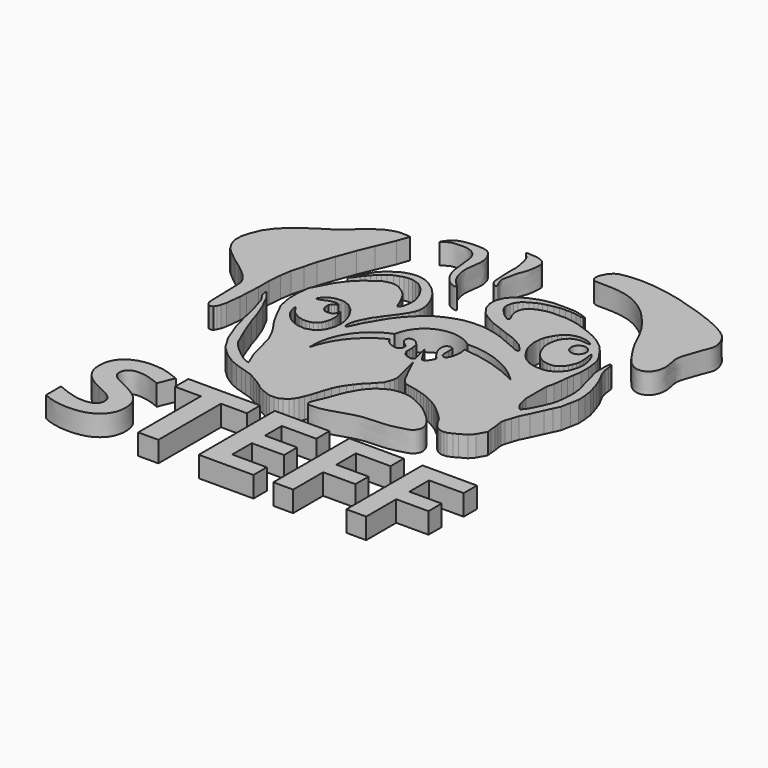
from build123d import *

# Parameters (mm, degrees)
F0_R         = 0.7148754106
F1_DEPTH     = 2
F2_TEXT_SIZE = 12.8132962143
F3_DEPTH     = 2


# Not quite as in the source:
# - Text() gives the source's letters only with a copy of the font that has no kerning and outlines rounded to 1/6400 em; it was checked with that copy


with BuildPart() as f1:
    # F0 (on Top) → F1 (new body)
    with BuildSketch(Plane.XY):
        Polygon((24.2907386273, 8.5276849568), (23.6116535962, 11.1627820879), (24.8693041503, 8.5963644087), (25.0527132303, 8.346952498), (25.2517424524, 8.1386491656), (25.4696086049, 8.0059850588), (25.712300092, 7.9455329105), (26.0382480919, 7.8855678439), (26.3718944043, 7.8116664663), (26.6574658453, 7.7494843863), (27.1523203701, 7.6115736738), (27.561949566, 7.478334941), (27.965053916, 7.3233088478), (28.3012557775, 7.1526789106), (28.7174619734, 6.9484477863), (29.083294794, 6.734599825), (29.4517893344, 6.4759417437), (29.7768972814, 6.1944676563), (30.1108527929, 5.9097232297), (30.4275006056, 5.6273424998), (30.7160790929, 5.3253171997), (30.9498113344, 5.0806938009), (31.1575550586, 4.7167097218), (31.3333831728, 4.4164536521), (31.5317050489, 4.1467623255), (31.7468166899, 3.954929697), (31.9705717266, 3.7988221738), (32.2670228779, 3.6963894963), (32.5457528234, 3.6963894963), (32.8103117645, 3.7337348331), (33.2356244326, 3.9057510439), (33.6025530184, 4.127406268), (34.2337685054, 4.4553116895), (34.6451625228, 4.9206055701), (35.1030383865, 5.7764222953), (35.0452120334, 6.2305437235), (35.0145325065, 6.7541487515), (34.9361580001, 7.2351241033), (34.886803478, 7.6227146201), (34.9578771205, 8.0304975484), (35.1350092745, 8.5627562235), (35.3541485965, 9.2212408781), (35.7608534396, 10.0460797548), (36.248870194, 11.1179118976), (36.5554206073, 11.7735937238), (36.8498107069, 12.3952152207), (37.0237194002, 13.3052840829), (37.1836354921, 14.1115276293), (37.134337691, 14.952889251), (37.0374396443, 15.7138481736), (36.8498107069, 16.3053733847), (36.6619750857, 16.906498), (36.4415954424, 17.4924607419), (36.1356697977, 18.0813653228), (35.888556391, 18.5570567846), (35.7323108402, 19.0970151623), (35.6707081445, 19.5807929325), (35.6309190392, 19.893264398), (35.5439911266, 20.0728083305), (35.3934951127, 20.0257822871), (35.3541485965, 18.992587924), (35.3976197821, 18.2506686842), (35.6607027352, 17.4087323248), (35.9177728508, 16.352175986), (36.1356697977, 15.6548470259), (36.2420044839, 14.8197803646), (36.2420044839, 14.1903264448), (36.1978299916, 13.4835708886), (36.0890701413, 12.796677649), (35.888556391, 12.194160372), (35.6456115842, 11.6420071572), (35.3640131652, 11.0622476786), (35.1376309991, 10.6370896101), (34.7761988164, 10.1604085924), (34.6406921744, 10.1180663332), (34.5081761479, 10.3389276192), (34.2337685054, 10.7001692558), (34.0774953365, 11.2002855167), (33.9554265588, 11.7979329079), (33.9554265588, 12.4641489238), (33.9554265588, 13.3207123727), (33.9554265588, 14.2623815543), (34.1256596148, 14.9280913174), (34.2337685054, 15.7283823937), (34.3045257032, 16.3797922432), (34.3799516559, 16.9626325369), (34.5074385405, 17.7104417235), (34.5074385405, 18.1742515415), (34.5074385405, 18.6049304903), (34.4467014074, 19.1184319556), (34.3787092705, 19.6089588158), (34.2337685054, 20.0728083305), (33.9935868979, 20.5351561308), (33.6651131511, 20.9820568562), (33.3983413875, 21.3733203709), (32.9359397292, 21.8890774995), (32.464645803, 22.2803428769), (31.9755636156, 22.6138047874), (31.4716597906, 22.8858546951), (30.7917307192, 23.1823699325), (30.0647059854, 23.4439208808), (29.4207148254, 23.6756000668), (28.7761632353, 23.8058827817), (28.0895289034, 23.8949786872), (27.538202703, 23.8949786872), (27.1113682538, 23.8949786872), (26.7201047391, 23.8949786872), (26.2932702899, 23.823838681), (25.8842222393, 23.7215775996), (25.4940543223, 23.5871449113), (25.1194797456, 23.3925599605), (24.8438157141, 23.1524650007), (24.6570762247, 22.9034796357), (24.5589371771, 22.509438917), (24.5589371771, 22.1156086773), (24.6831804903, 21.6857026522), (24.7969844564, 21.4666308677), (24.9062236398, 21.2563462555), (24.9062236398, 21.1131349206), (24.8109105975, 21.021023119), (24.6842466295, 21.0665911436), (24.4121458381, 21.242024377), (24.1257250309, 21.4711613953), (23.8249823451, 21.7719040811), (23.5651400528, 22.0967382025), (23.3939066529, 22.4263612181), (23.3939066529, 22.7287001908), (23.4363881231, 23.0534564958), (23.5403869301, 23.342538625), (23.7226802856, 23.6493237317), (23.9805597812, 23.8983109593), (24.382356189, 24.1568095487), (24.6950193107, 24.3192325799), (24.9631647021, 24.4585294276), (25.3410916775, 24.5830230415), (25.7301535457, 24.6850401163), (26.2492913753, 24.7960276902), (26.746949181, 24.8712133616), (27.2768270224, 24.8998552561), (27.8496704996, 24.8998552561), (28.3222645521, 24.8568914831), (28.8235023618, 24.7540798282), (29.1257899468, 24.7540798282), (29.1638504714, 24.8598754406), (28.5766869783, 25.0711105764), (27.9537215829, 25.2035818994), (27.3271705955, 25.2300128341), (26.6277603805, 25.2300128341), (25.8872099221, 25.2300128341), (25.2358000726, 25.1134447753), (24.6392469853, 24.9557346106), (23.9192657173, 24.6677435935), (23.3912821859, 24.3934653699), (22.904438898, 23.9957626909), (22.5187186152, 23.5871449113), (22.1901535988, 22.8337235749), (22.1901535988, 22.1508350223), (22.3913134389, 21.4811542993), (22.9124389589, 20.7325294614), (23.5034003854, 20.312288776), (24.3307463825, 19.8657847941), (25.2762846649, 19.5112079382), (26.195557788, 19.1566310823), (27.1148309112, 18.8414528966), (28.0735008419, 18.2898882776), (28.6644622684, 17.6595300436), (28.6644622684, 17.4625422806), (28.4018144011, 17.4625422806), (28.0341040343, 17.6332648844), (27.5876000524, 17.8302526474), (26.9703734666, 18.0797688663), (26.3925455511, 18.3424185961), (25.65712668, 18.605068326), (24.8166490346, 18.7889225781), (24.1206269711, 18.8939832151), (23.2276190072, 18.8939832151), (22.3477426916, 18.7889225781), (21.5991921723, 18.5788031667), (20.942568779, 18.3161534369), (20.2356303337, 17.9612244696), (19.5574704558, 17.4891503396), (18.94024387, 16.8775692582), (18.3886792511, 16.29973948), (17.8765133023, 15.6431160867), (17.3677299172, 14.8263750598), (17.0370518032, 14.2229637131), (16.7094636708, 13.7018356472), (16.4351854473, 13.0847096443), (16.2500478327, 12.7144344151), (16.1197669804, 12.5061682631), (15.9746445923, 12.5061682631), (15.9414857626, 12.6047236845), (15.9414857626, 12.9818553105), (16.0437058657, 13.4173221886), (16.1877013743, 13.8561669737), (16.434552148, 14.3018681556), (16.6196897626, 14.699571766), (16.9143974781, 15.0882480666), (17.1527792951, 15.4448095709), (17.4903795123, 15.904225409), (17.8496371955, 16.4013300091), (18.1257128716, 16.793359071), (18.3797031641, 17.1909090132), (18.60056445, 17.616065219), (18.7287908047, 18.0798731744), (18.7287908047, 18.5411386192), (18.6502356082, 19.0139841288), (18.4901729226, 19.4897260517), (18.3062069118, 19.9071634561), (18.0687734729, 20.3393351903), (17.7815575153, 20.7519363612), (17.461432144, 21.1076308042), (17.1032305807, 21.4480049908), (16.6780743748, 21.7516887933), (16.3688678294, 21.9559855759), (15.9713178873, 22.1326742321), (15.5075099319, 22.2375839949), (15.1099609211, 22.2872775048), (14.6461520344, 22.2431048751), (14.1713013873, 22.1326742321), (13.7847941369, 21.9780709594), (13.3872451261, 21.7461679131), (13.0614750087, 21.5087421238), (12.6804895699, 21.2050583214), (12.3034892604, 20.8377465606), (11.8868350983, 20.1465655118), (11.5168923512, 19.516505301), (11.1311545422, 18.8449039694), (11.2187303603, 18.771706149), (11.5279359743, 19.1416479647), (11.7989871651, 19.516505301), (12.0384553447, 19.8146682233), (12.3034892604, 20.1349165291), (12.6182157546, 20.4662084579), (12.9119114889, 20.7217949708), (13.2593411217, 20.9636443443), (13.6547806244, 21.2389138865), (14.1084849047, 21.4004018793), (14.4286891446, 21.5143729001), (14.8372817785, 21.5640664101), (15.201702714, 21.5640664101), (15.5661236495, 21.4702002704), (15.9802380949, 21.3155969977), (16.3897592574, 21.0091285408), (16.6838439588, 20.6882080435), (16.9931514671, 20.243871172), (17.249884792, 19.776975354), (17.4682307988, 19.008398056), (17.4682307988, 18.3950569481), (17.3413343728, 17.7605655044), (17.1527792951, 17.5220274957), (17.0370518032, 17.4891503396), (16.912657733, 17.667849112), (16.7705746947, 18.0670347203), (16.5224865601, 18.5686041272), (16.1992479116, 19.1564466804), (15.7762542367, 19.5794403553), (15.3321102262, 19.8755376041), (15.0360139087, 20.0447347015), (14.6341696382, 20.1482789205), (14.2209337805, 20.1482789205), (13.6408779873, 19.9834902043), (13.1381272476, 19.6335201961), (12.4223483726, 19.1352590919), (11.7989871651, 18.5574293137), (11.3192200661, 17.9664678872), (10.8595835045, 17.2967128456), (10.4262121022, 16.4562352002), (9.9797081202, 15.6420208514), (9.8468763754, 14.5015092567), (9.8468763754, 13.4440232068), (10.0920091452, 12.1402390962), (10.7457740232, 10.8184972778), (11.3288797438, 9.7580598667), (11.7989871651, 9.0827252716), (12.2325560078, 8.4165092558), (12.7189997584, 7.4330470525), (12.9833715037, 6.5024592914), (13.2265929133, 5.5824466981), (13.4197808802, 4.750484135), (14.0289058909, 3.304582322), (13.333641924, 3.6060682032), (12.6691423357, 4.0982901119), (11.9061982259, 4.750484135), (11.3293491304, 5.4122628644), (10.6122841348, 7.0427347797), (9.9340314046, 8.8061923161), (9.6277336048, 9.7929947206), (9.1117341071, 11.1345937476), (8.4279282019, 12.4762374908), (7.9319133823, 13.1022745853), (7.804713212, 13.1167639047), (7.9449221191, 12.5772664323), (8.3759939298, 11.9222681969), (8.862381801, 10.3419721127), (9.1928914189, 8.8791605085), (9.5785651356, 7.4076233432), (10.3000886738, 5.5316616781), (11.0682053491, 4.2288983241), (11.9425226003, 3.3970240038), (12.8638958558, 2.7919441927), (13.5361524299, 2.491829684), (14.148385264, 2.2997565102), (14.6885914728, 2.1316925995), (15.3428409249, 1.9216125365), (15.8410295844, 1.651509665), (16.4112485945, 1.3093793532), (16.901128231, 0.9802823328), (17.2268431634, 0.7096152985), (17.7006591111, 0.48602483), (18.159776926, 0.2906816371), (18.5862127692, 0.1488179405), (19.0066304058, 0.1488179405), (19.4182936102, 0.204862401), (19.7184178978, 0.3563134233), (20.102272972, 0.6089386869), (20.3555040061, 0.9136715089), (20.5445941538, 1.2202296639), (20.7265391946, 1.66916952), (20.9399685264, 2.1973256953), (21.1050435901, 2.7211178094), (21.302357316, 3.3580199815), (21.5112250298, 3.9624199271), (21.7900946736, 4.5490162447), (22.103626281, 5.0381072797), (22.4218014628, 5.4770857096), (22.8315256536, 5.9701390564), (23.2227928936, 6.3579040579), (23.6271154135, 6.7892442457), (23.9983685315, 7.2086052969), (24.1765435785, 7.6831914485), (24.2907386273, 8.0683119595), align=None)
        Polygon((11.4993210882, 14.6436599655), (11.4807495847, 14.6839478984), (11.7608709261, 15.1338391006), (12.1343657374, 15.3884943575), (12.6351881772, 15.5667532235), (13.1190326065, 15.6091963872), (13.5179935023, 15.5667532235), (13.9678847045, 15.3884952888), (14.2989363521, 15.1338391006), (14.6214999259, 14.8409856483), (14.8464459926, 14.5269101486), (15.1265664026, 14.0600418672), (15.2963371947, 13.6525938287), (15.4321538284, 13.1984576583), (15.5191710219, 12.5772664323), (15.4321538284, 11.9066741318), (15.2305616066, 11.2955011427), (14.9249751121, 10.8371209353), (14.4478578531, 10.4954016644), (13.8052644282, 10.303223896), (13.1184505299, 10.3686060756), (12.5454757363, 10.5638420209), (12.1337827295, 10.8184972778), (11.7608709261, 11.1570615731), (11.4165032282, 11.5569978952), (11.234426235, 11.9939806813), (11.1311545422, 12.3392948731), (11.1311545422, 12.6277012751), (11.3157930783, 12.3699041891), (11.4410180856, 12.1611954273), (11.5607800518, 11.9939806813), (11.7608709261, 11.8123194273), (11.9937377027, 11.6682782417), (12.1969040271, 11.5426084545), (12.4516179785, 11.4302448928), (12.7757415175, 11.3492142409), (13.1388790905, 11.3252056763), (13.4509988129, 11.3702220842), (13.7762400245, 11.4674906336), (14.0457884462, 11.6605456706), (14.2312953249, 11.9074266404), (14.3693480641, 12.1925352141), (14.4478578531, 12.4922143295), (14.5048173144, 12.8190219402), (14.5048173144, 13.1246084347), (14.4478578531, 13.4301949292), (14.3632018443, 13.7132630232), (14.2473119399, 14.1007692949), (14.2034748569, 13.9395063743), (14.1482995823, 13.7230493128), (13.9678847045, 13.5243312602), (13.7666308612, 13.4404751088), (13.4869674221, 13.4246200323), (13.2450452074, 13.4755503386), (13.0654336696, 13.5866501668), (12.9474079253, 13.7833601329), (12.8560017639, 14.0889990152), (12.8560017639, 14.3917575479), (12.9880212729, 14.6051892645), (13.1649551913, 14.7668998688), (13.3470012526, 14.8213436345), (13.492080383, 14.8213436345), (13.3693711012, 14.9926734984), (13.2219772786, 15.0340022519), (12.9998922348, 15.0340022519), (12.7477962524, 15.0340022519), (12.5125863395, 14.9636589922), (12.2378331184, 14.8491779601), (11.8866462507, 14.7028494296), (11.6887317845, 14.6436599655), align=None, mode=Mode.SUBTRACT)
        with BuildLine():
            ThreePointArc((21.2132986635, 12.1578685939), (20.4473145006, 12.3519211299), (19.9188143015, 12.9393525422))
            ThreePointArc((19.9188143015, 12.9393525422), (17.4443393612, 10.9808286692), (16.0302296281, 8.1596346572))
            Line((16.0302296281, 8.1596346572), (16.0302296281, 8.8887438178))
            ThreePointArc((16.0302296281, 8.8887438178), (17.1309249273, 11.8998701151), (19.6871741574, 13.8348123865))
            ThreePointArc((19.6871741574, 13.8348123865), (21.7523585958, 16.4088665275), (25.0181499869, 15.9341581166))
            ThreePointArc((25.0181499869, 15.9341581166), (28.3436366182, 15.3365141693), (31.1502087861, 13.4552400559))
            ThreePointArc((31.1502087861, 13.4552400559), (28.3497777615, 14.5861581292), (25.3769401461, 15.1187237352))
            ThreePointArc((25.3769401461, 15.1187237352), (25.4422622613, 14.1382532612), (25.1048468053, 13.2153555751))
            Line((25.1048468053, 13.2153555751), (24.8670708388, 13.2130132988))
            Line((24.8670708388, 13.2130132988), (24.6725827456, 13.3162793097))
            Line((24.6725827456, 13.3162793097), (24.6054362506, 13.559114188))
            Line((24.6054362506, 13.559114188), (24.6054362506, 13.7894693762))
            Line((24.6054362506, 13.7894693762), (24.6054362506, 14.1558581963))
            Line((24.6054362506, 14.1558581963), (24.526713416, 14.7497151047))
            Line((24.526713416, 14.7497151047), (24.2627672851, 14.822665602))
            Line((24.2627672851, 14.822665602), (23.9884052426, 14.7470263764))
            Line((23.9884052426, 14.7470263764), (23.8182302564, 14.4827486947))
            Line((23.8182302564, 14.4827486947), (23.8182302564, 14.0603547916))
            Line((23.8182302564, 14.0603547916), (23.9779874682, 13.5713601485))
            Line((23.9779874682, 13.5713601485), (24.3312194943, 13.0185233429))
            Line((24.3312194943, 13.0185233429), (24.523390457, 12.8111243248))
            Line((24.523390457, 12.8111243248), (24.6403124183, 12.662248686))
            Line((24.6403124183, 12.662248686), (24.6241055429, 12.5214504078))
            Line((24.6241055429, 12.5214504078), (24.4701392949, 12.2323455289))
            Line((24.4701392949, 12.2323455289), (24.3034362793, 11.9946226478))
            Line((24.3034362793, 11.9946226478), (24.1066366434, 11.8316644803))
            Line((24.1066366434, 11.8316644803), (23.8820519298, 11.8430582806))
            Line((23.8820519298, 11.8430582806), (22.9702237631, 13.3162793097))
            Line((22.9702237631, 13.3162793097), (23.3807861805, 11.7220170796))
            Line((23.3807861805, 11.7220170796), (23.2279766351, 11.4827072248))
            Line((23.2279766351, 11.4827072248), (22.9779239744, 11.5112746134))
            Line((22.9779239744, 11.5112746134), (22.7324981242, 11.5678431466))
            Line((22.7324981242, 11.5678431466), (22.4511884153, 11.7069706321))
            Line((22.4511884153, 11.7069706321), (22.2798530012, 11.911990121))
            Line((22.2798530012, 11.911990121), (22.1501979977, 12.1550420299))
            Line((22.1501979977, 12.1550420299), (22.1571419388, 12.5495754182))
            Line((22.1571419388, 12.5495754182), (22.1571419388, 12.8817595541))
            Line((22.1571419388, 12.8817595541), (22.0159050077, 13.5255521163))
            Line((22.0159050077, 13.5255521163), (21.7704791576, 13.7960957363))
            Line((21.7704791576, 13.7960957363), (21.4602295309, 13.9741916209))
            Line((21.4602295309, 13.9741916209), (21.1522914469, 13.9951081946))
            Line((21.1522914469, 13.9951081946), (20.9300220013, 13.8493236154))
            Line((20.9300220013, 13.8493236154), (20.8744574338, 13.5989040136))
            Line((20.8744574338, 13.5989040136), (20.9601242095, 13.3466133848))
            Line((20.9601242095, 13.3466133848), (21.138401702, 13.1408013403))
            Line((21.138401702, 13.1408013403), (21.4046649635, 12.9534667358))
            Line((21.4046649635, 12.9534667358), (21.5806290507, 12.7594145015))
            Line((21.5806290507, 12.7594145015), (21.5806290507, 12.4768838286))
            Line((21.5806290507, 12.4768838286), (21.4347653091, 12.2795756906))
            Line((21.4347653091, 12.2795756906), (21.2132986635, 12.1578685939))
        make_face(mode=Mode.SUBTRACT)
        Polygon((32.2024236749, 21.6673035175), (32.179441303, 21.6673035175), (31.8553186953, 21.6673035175), (31.6520147026, 21.7021815479), (31.3518978655, 21.7141862959), (31.1253126711, 21.6976795346), (30.8672133833, 21.6466598213), (30.6331254542, 21.5551257133), (30.4485540837, 21.4485842735), (30.3285084665, 21.3360413909), (30.1994588226, 21.196488291), (30.0794132054, 21.0584364831), (29.9531836063, 20.8845473826), (29.876653105, 20.7029785961), (29.8181306571, 20.5034017563), (29.7716129571, 20.3068275005), (29.7296587378, 20.0684703887), (29.7101512551, 19.8403839022), (29.7101512551, 19.6099672467), (29.7312997282, 19.3923842162), (29.7497604042, 19.2497763783), (29.7910254449, 19.1034711897), (29.8382937908, 18.9721714705), (29.9531836063, 18.6746716499), (30.0661027431, 18.4345804155), (30.2242137853, 18.1606703597), (30.3860846907, 17.9432407022), (30.5855646729, 17.7480056882), (30.8105107397, 17.5527688116), (31.0566779226, 17.4084641039), (31.3004666664, 17.3057081451), (31.5968194016, 17.2535458766), (31.9516181814, 17.2232011107), (32.3257111013, 17.2768924385), (32.6243907518, 17.4493014094), (32.8647308052, 17.6673643291), (33.0939218402, 17.9771948606), (33.227863254, 18.2949711665), (33.362194065, 18.6136713179), (33.4231950064, 18.9602397545), (33.4231950064, 19.3628575653), (33.3946980536, 19.708763808), (33.3308726549, 20.182909444), (33.3308726549, 20.4860251397), (33.4231950064, 20.3599780798), (33.6099788547, 20.0838726014), (33.7690375745, 19.708763808), (33.8740795851, 19.3726010621), (33.9617356658, 18.7977515161), (33.914945481, 18.2506686842), (33.7690375745, 17.6800843328), (33.6076992835, 17.2973088741), (33.3014242351, 16.8933086097), (33.0149382353, 16.6641175747), (32.6690301299, 16.4476614445), (32.3837674713, 16.3267005017), (32.0691242814, 16.2773840129), (31.7510031164, 16.263877973), (31.4508862793, 16.263877973), (31.1807841063, 16.2998922169), (30.9116253781, 16.3472679559), (30.6050814688, 16.4384189993), (30.3304772824, 16.5839754045), (30.1233995706, 16.708523035), (29.9004749988, 16.8775235037), (29.7210048884, 17.0521531254), (29.5469388366, 17.2532293946), (29.3863769621, 17.470812425), (29.2678326368, 17.6523812115), (29.1584187551, 17.8419287727), (29.0295065137, 18.0652551057), (28.9070916571, 18.3539465347), (28.8274753839, 18.6846721917), (28.7764556706, 19.0177988261), (28.7404414266, 19.2668940872), (28.7404414266, 19.5399969816), (28.7760427729, 19.9562570463), (28.8724050523, 20.3330893235), (28.9996804032, 20.6350503802), (29.1660893708, 20.9401287138), (29.3881744146, 21.2942622602), (29.6012554318, 21.5373560786), (29.8684542652, 21.7686625684), (30.1711949092, 21.9434156953), (30.5605319106, 22.0650732611), (31.0262441635, 22.1273452044), (31.4108729362, 22.0767054707), (31.7305819401, 21.9949505622), (32.1111753583, 21.8178052455), align=None, mode=Mode.SUBTRACT)
        with Locations((32.1084111929, 20.4434879124)):
            Circle(F0_R, mode=Mode.SUBTRACT)
    extrude(amount=F1_DEPTH)


with BuildPart() as f1b:
    # F0 (on Top) → F1, piece 2 (new body)
    with BuildSketch(Plane.XY):
        with BuildLine():
            add(Edge.make_bspline(
                [(21.6533839703, 0.9376612725), (21.5461532449, 1.1311018136), (22.0344466379, 2.0685321705), (22.4233865431, 3.1960527643), (22.7976823898, 4.1928911727), (23.4322410303, 5.3064863476), (24.0741523461, 5.9862297193), (24.9213836542, 6.4999262835), (25.5587741255, 6.7000867161), (26.749762737, 6.7702439862), (27.9176928338, 6.2376283208), (28.8198512588, 5.7654688033), (29.6107819403, 5.0857277809), (30.2381366471, 4.5356280251), (30.7263070916, 3.8476718611), (30.9750342426, 3.1452677218), (30.5835102235, 2.3943301946), (29.710791279, 2.1818872726), (28.6218613791, 1.895754702), (27.3538366614, 1.8417881518), (26.2622725948, 1.8209466564), (25.1013141845, 1.4925906791), (24.2392848072, 1.2327041384), (23.160959641, 0.8574094608), (22.3444714616, 0.790687727), (21.7348617966, 0.7906780755), (21.6533839703, 0.9376612725)],
                knots=[0, 0, 0, 0, 0.0438321528, 0.0917117069, 0.134904964, 0.1818612444, 0.2228157202, 0.2634959627, 0.2977575359, 0.3425918062, 0.3900760191, 0.4325789289, 0.4749537877, 0.5133887574, 0.5515986715, 0.5867264002, 0.6223953051, 0.6611041658, 0.7059206258, 0.7530279547, 0.7971544854, 0.8425262759, 0.8828675863, 0.9269997768, 0.9666947274, 1, 1, 1, 1], degree=3))
        make_face()
    extrude(amount=F1_DEPTH)


with BuildPart() as f1c:
    # F0 (on Top) → F1, piece 3 (new body)
    with BuildSketch(Plane.XY):
        Polygon((10.3225391358, 25.7849916816), (10.7130110264, 26.9054751843), (10.3810051279, 26.9496183768), (9.9722283454, 26.9686307203), (9.4923535362, 26.9548874348), (8.9554619044, 26.7985071987), (8.3642359823, 26.5584159642), (7.6800277457, 26.0781962425), (6.9777597673, 25.531988591), (6.3415174372, 24.9197557569), (5.6360246401, 24.3455377762), (4.846948199, 23.8633528352), (3.1822551973, 22.7532535791), (2.4919921998, 22.1590269357), (1.8679589467, 21.5046327781), (1.3222009086, 20.7276864662), (1.0364311747, 20.0472828001), (0.8728378755, 19.5575063688), (0.7451109813, 19.0589597071), (0.7146475837, 18.4794794768), (0.7926773396, 18.0983357131), (0.9277287754, 17.6481641829), (1.3414554996, 16.9711168855), (1.8028729828, 16.5448077023), (2.7450982016, 15.7723538578), (3.6151711829, 15.1611799374), (4.1467333212, 14.729898423), (4.5541818254, 14.3946027383), (4.9276766367, 14.0041308478), (5.2290190943, 13.6051708832), (5.4014078283, 13.1647829058), (5.4376195185, 12.7685843036), (5.5297608487, 9.5512820408), (5.5658370256, 9.1565661132), (5.6634549983, 8.9464746416), (5.7838540806, 8.7997708639), (5.9732859954, 8.7512386963), (6.1366898008, 8.7724607438), (6.2449183315, 8.8276360184), (6.3986195855, 9.0623761355), (6.5266615711, 9.3672377989), (6.6582337022, 9.8807932809), (6.8224286661, 11.3222431391), (6.8554407917, 12.032023631), (6.9268648513, 13.3906649426), (6.9268648513, 14.646965079), (7.0286970586, 15.9067641944), (7.1907588281, 16.975171864), (7.5088799931, 18.1456170976), (7.8266048804, 19.3222220987), (8.3528934047, 20.884109661), (8.9983306825, 22.6272642612), (9.6095036715, 24.0872893482), align=None)
    extrude(amount=F1_DEPTH)


with BuildPart() as f1d:
    # F0 (on Top) → F1, piece 4 (new body)
    with BuildSketch(Plane.XY):
        with BuildLine():
            add(Edge.make_bspline(
                [(12.9611995071, 27.6486929506), (12.9265816392, 27.6806340367), (13.409266983, 28.4060815464), (14.1391738196, 28.7875023851), (15.1670985556, 28.9129633362), (16.6962123952, 28.9130324962), (17.2309082519, 28.120901091), (17.5655747598, 27.2347063276), (17.2669091669, 25.8609796459), (17.2619594602, 24.7553564461), (17.6767481745, 23.6780876745), (18.0169875926, 23.2595467722), (18.7905812918, 22.5907394254), (17.8162037274, 22.8119645619), (17.2353272406, 23.4066244997), (16.772719512, 24.2254844379), (16.6081930146, 25.1865888603), (16.4897872647, 26.3057501391), (16.4289246388, 27.2071980229), (15.9885310343, 27.8903199812), (15.1699376584, 28.219373191), (14.2303607047, 28.173022289), (13.5172526507, 28.1012783461), (12.9922047839, 27.6200851166), (12.9611995071, 27.6486929506)],
                knots=[0, 0, 0, 0, 0.0413466402, 0.0868576102, 0.1358895009, 0.1934344759, 0.2375944162, 0.2834447771, 0.3395217085, 0.3909380912, 0.4405849392, 0.4790406032, 0.5170802349, 0.5532951469, 0.5990031346, 0.6446982846, 0.692066406, 0.7431589958, 0.7885099814, 0.8299872204, 0.8739776978, 0.9200161018, 0.9629681403, 1, 1, 1, 1], degree=3))
        make_face()
    extrude(amount=F1_DEPTH)


with BuildPart() as f1e:
    # F0 (on Top) → F1, piece 5 (new body)
    with BuildSketch(Plane.XY):
        with BuildLine():
            add(Edge.make_bspline(
                [(19.1949084401, 30.2752405405), (19.2299629828, 30.3629572786), (19.9991069873, 30.3036361919), (20.6810365577, 30.2045196175), (21.273984256, 29.7318252679), (21.1991415403, 28.9326127705), (21.1072048676, 28.0833699025), (20.7108312486, 27.2685849641), (20.6061108666, 26.4633932944), (20.3954914866, 25.7429724616), (20.5552500067, 25.3389111635), (20.9889152633, 24.4641505379), (20.1383334147, 24.9605042962), (20.156471754, 25.8106926079), (20.0366694834, 26.8970667416), (20.1308694593, 27.8114132973), (19.9877284444, 28.6863813564), (19.8281819653, 29.3955025372), (19.5956594338, 29.8796229102), (19.1656944198, 30.202138501), (19.1949084401, 30.2752405405)],
                knots=[0, 0, 0, 0, 0.0545707873, 0.112618597, 0.1644780812, 0.2203112256, 0.280705754, 0.3418799886, 0.4009480961, 0.4548920345, 0.5006596675, 0.5517953204, 0.5989845328, 0.6590858936, 0.7270591869, 0.7894129844, 0.850191985, 0.9047490551, 0.9545213839, 1, 1, 1, 1], degree=3))
        make_face()
    extrude(amount=F1_DEPTH)


with BuildPart() as f1f:
    # F0 (on Top) → F1, piece 6 (new body)
    with BuildSketch(Plane.XY):
        with BuildLine():
            add(Edge.make_bspline(
                [(26.4925137162, 31.8238697946), (26.2542845134, 31.6692354501), (25.9147245809, 31.1976317374), (25.700804084, 30.6083268194), (25.7631752123, 29.9493769725), (26.8228706758, 29.9081628319), (27.8449163362, 29.9491625629), (29.461522842, 29.7149935833), (30.6924802322, 29.1044852219), (31.8344768736, 28.2986303406), (32.7784942215, 27.242139577), (33.6593554272, 26.1465713274), (34.3006318106, 24.8987351945), (34.847213988, 23.6499967403), (35.7178369576, 22.3079745175), (36.6041041875, 21.0550466969), (37.6305826087, 20.5872272471), (38.5766423237, 20.9616967363), (38.9669497769, 21.8350159201), (38.9886804985, 22.7907449894), (38.6047081472, 23.9038143438), (39.0804031666, 25.1666511687), (39.4148319278, 26.2765423367), (39.958468497, 27.2567452549), (39.4369477463, 28.669073313), (38.6170003084, 29.3980288063), (37.2281612417, 30.1159194179), (35.7698358355, 30.6849153765), (34.4510778872, 31.1082530647), (32.8300933021, 31.6107100311), (31.4926098955, 31.8850752191), (30.1949395178, 32.1251264901), (28.6745478952, 32.2159448639), (27.4232406311, 32.1046859432), (26.7436157537, 31.9868598836), (26.4925137162, 31.8238697946)],
                knots=[0, 0, 0, 0, 0.0253262569, 0.0473296945, 0.0668451636, 0.0928984122, 0.1218263983, 0.1565980223, 0.1890418557, 0.2213383338, 0.2540962653, 0.2867645686, 0.3191919175, 0.351327877, 0.386382581, 0.4204773655, 0.4483850578, 0.4744152861, 0.5004403442, 0.527137413, 0.5564625754, 0.5879963093, 0.6178362365, 0.6461962967, 0.6783758844, 0.7072225338, 0.7414389271, 0.7759953311, 0.8085879738, 0.844353577, 0.8765907492, 0.9081641096, 0.9422042534, 0.9733052261, 1, 1, 1, 1], degree=3))
        make_face()
    extrude(amount=F1_DEPTH)


with BuildPart() as f3:
    # F2 (on Top) → F3 (new body)
    with BuildSketch(Plane.XY):
        with Locations((4.8455442302, -10.722522682)):
            Text('STEFF', F2_TEXT_SIZE, font='Open Sans', font_style=FontStyle.BOLD, text_align=(TextAlign.LEFT, TextAlign.BOTTOM))
    extrude(amount=F3_DEPTH)


solid = Compound([f1.part, f1b.part, f1c.part, f1d.part, f1e.part, f1f.part, f3.part])
